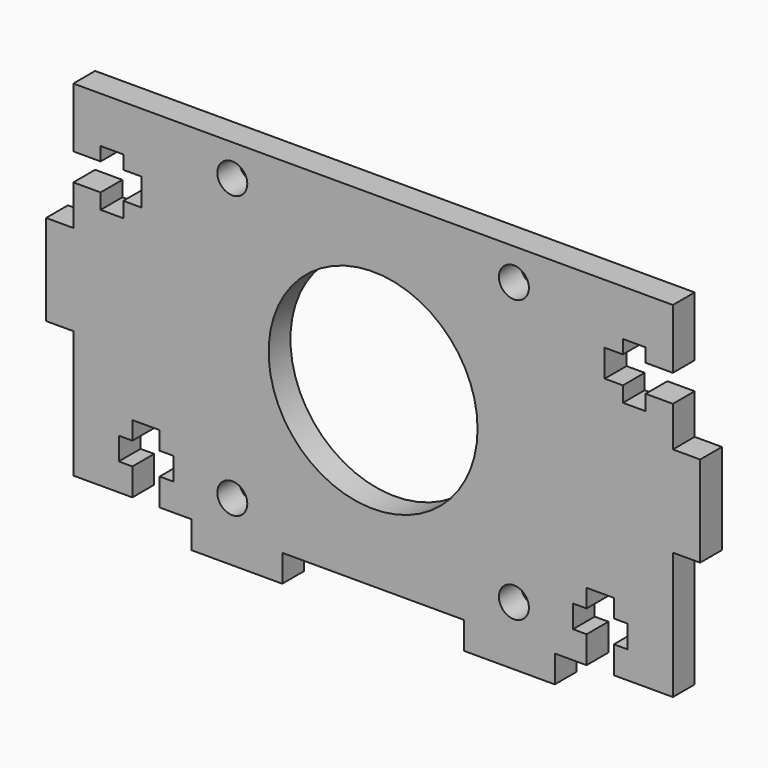
from build123d import *

# Parameters (mm, degrees)
F0_R     = 1.65
F0_R_2   = 11.5
F1_DEPTH = 3
F3_DEPTH = 3


# Not quite as in the source:
# - a feature names something its author has since deleted; it is built from what else it names


with BuildPart() as f1:
    # F0 (on Front) → F1 (new body)
    with BuildSketch(Plane.XZ):
        Polygon((33, 5), (33, 19), (-33, 19), (-33, 5), (-36, 5), (-36, -5), (-33, -5), (-33, -19), (-20, -19), (-20, -22), (-10, -22), (-10, -19), (0, -19), (10, -19), (10, -22), (20, -22), (20, -19), (33, -19), (33, -5), (36, -5), (36, 5), align=None)
        with Locations((-15.5, -15.5)):
            Circle(F0_R, mode=Mode.SUBTRACT)
        with Locations((15.5, -15.5)):
            Circle(F0_R, mode=Mode.SUBTRACT)
        with Locations((-15.5, 15.5)):
            Circle(F0_R, mode=Mode.SUBTRACT)
        Circle(F0_R_2, mode=Mode.SUBTRACT)
        with Locations((15.5, 15.5)):
            Circle(F0_R, mode=Mode.SUBTRACT)
    extrude(amount=F1_DEPTH)

    # F2 (on face) → F3 (cut, through all)
    with BuildSketch(Plane.XZ.offset(3)):
        Polygon((23.5, -16), (23.5, -19), (26.5, -19), (26.5, -16), (28, -16), (28, -13.5), (26.5, -13.5), (26.5, -11.5), (23.5, -11.5), (23.5, -13.5), (22, -13.5), (22, -16), align=None)
        Polygon((-26.5, -19), (-23.5, -19), (-23.5, -16), (-22, -16), (-22, -13.5), (-23.5, -13.5), (-23.5, -11.5), (-26.5, -11.5), (-26.5, -13.5), (-28, -13.5), (-28, -16), (-26.5, -16), align=None)
        Polygon((30, 9.4201220199), (33, 9.4201220199), (33, 11), (33, 12.4201220199), (30, 12.4201220199), (30, 13.9201220199), (27.5, 13.9201220199), (27.5, 12.4201220199), (25.5, 12.4201220199), (25.5, 9.4201220199), (27.5, 9.4201220199), (27.5, 7.7319853008), (30, 7.7319853008), align=None)
        Polygon((-30, 12.4201220199), (-33, 12.4201220199), (-33, 11), (-33, 9.4201220199), (-30, 9.4201220199), (-30, 7.7319853008), (-27.5, 7.7319853008), (-27.5, 9.4201220199), (-25.5, 9.4201220199), (-25.5, 12.4201220199), (-27.5, 12.4201220199), (-27.5, 13.9201220199), (-30, 13.9201220199), align=None)
    extrude(amount=-F3_DEPTH, mode=Mode.SUBTRACT)


solid = f1.part
